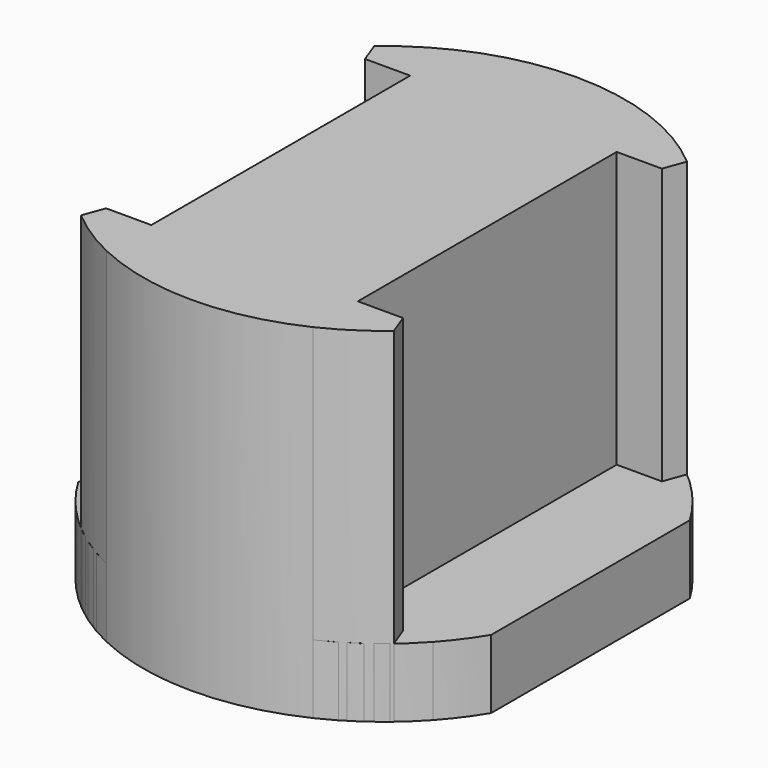
from build123d import *

# Parameters (mm, degrees)
F1_DEPTH    = 5
F0_W        = 15
F0_H        = 23.5
F2_DEPTH    = 25
F3_T1_DEPTH = 36.3750267574
F4_DEPTH    = 15


# Not quite as in the source:
# - a fillet or chamfer that OpenCascade refuses, or shapes differently, is made with other operations: its cross-section is extruded or revolved along the edge and cut away or added
# - a feature names something its author has since deleted; it is built from what else it names


with BuildPart() as f1:
    # F0 (on Top) → F1 (new body)
    with BuildSketch(Plane.XY):
        with BuildLine():
            Line((15, -9.0138781887), (15, 9.0138781887))
            ThreePointArc((15, 9.0138781887), (14.0511141288, 10.4314999755), (12.9687123493, 11.75))
            Line((12.9687123493, 11.75), (7.5, 11.75))
            Line((7.5, 11.75), (7.5, -11.75))
            Line((7.5, -11.75), (12.9687123493, -11.75))
            ThreePointArc((12.9687123493, -11.75), (14.0511141288, -10.4314999755), (15, -9.0138781887))
        make_face()
        with BuildLine():
            ThreePointArc((7.5, -15.8113883008), (10.4338758399, -14.0493499834), (12.9687123493, -11.75))
            Line((12.9687123493, -11.75), (7.5, -11.75))
            Line((7.5, -11.75), (7.5, -15.8113883008))
        make_face()
        with BuildLine():
            Line((7.5, 11.75), (12.9687123493, 11.75))
            ThreePointArc((12.9687123493, 11.75), (10.4338758399, 14.0493499834), (7.5, 15.8113883008))
            Line((7.5, 15.8113883008), (7.5, 11.75))
        make_face()
    extrude(amount=F1_DEPTH)


with BuildPart() as f1b:
    # F0 (on Top) → F1, piece 2 (new body)
    with BuildSketch(Plane.XY):
        with BuildLine():
            Line((-7.5, -11.75), (-7.5, 11.75))
            Line((-7.5, 11.75), (-12.9687123493, 11.75))
            ThreePointArc((-12.9687123493, 11.75), (-14.0511141288, 10.4314999755), (-15, 9.0138781887))
            Line((-15, 9.0138781887), (-15, -9.0138781887))
            ThreePointArc((-15, -9.0138781887), (-14.0511141288, -10.4314999755), (-12.9687123493, -11.75))
            Line((-12.9687123493, -11.75), (-7.5, -11.75))
        make_face()
        with BuildLine():
            Line((-7.5, 11.75), (-7.5, 15.8113883008))
            ThreePointArc((-7.5, 15.8113883008), (-10.4338758399, 14.0493499834), (-12.9687123493, 11.75))
            Line((-12.9687123493, 11.75), (-7.5, 11.75))
        make_face()
        with BuildLine():
            ThreePointArc((-12.9687123493, -11.75), (-10.4338758399, -14.0493499834), (-7.5, -15.8113883008))
            Line((-7.5, -15.8113883008), (-7.5, -11.75))
            Line((-7.5, -11.75), (-12.9687123493, -11.75))
        make_face()
    extrude(amount=F1_DEPTH)


with BuildPart() as f2:
    # F0 (on Top) → F2 (new body)
    with BuildSketch(Plane.XY):
        Rectangle(F0_W, F0_H)
        Polygon((-5.6291651246, 3.25), (0, 6.5), (5.6291651246, 3.25), (5.6291651246, -3.25), (0, -6.5), (-5.6291651246, -3.25), align=None, mode=Mode.SUBTRACT)
        with BuildLine():
            ThreePointArc((-12.9687123493, -11.75), (-10.4338758399, -14.0493499834), (-7.5, -15.8113883008))
            Line((-7.5, -15.8113883008), (-7.5, -11.75))
            Line((-7.5, -11.75), (-12.9687123493, -11.75))
        make_face()
        with BuildLine():
            Line((-7.5, 11.75), (-7.5, 15.8113883008))
            ThreePointArc((-7.5, 15.8113883008), (-10.4338758399, 14.0493499834), (-12.9687123493, 11.75))
            Line((-12.9687123493, 11.75), (-7.5, 11.75))
        make_face()
        with BuildLine():
            Line((7.5, 11.75), (12.9687123493, 11.75))
            ThreePointArc((12.9687123493, 11.75), (10.4338758399, 14.0493499834), (7.5, 15.8113883008))
            Line((7.5, 15.8113883008), (7.5, 11.75))
        make_face()
        with BuildLine():
            ThreePointArc((7.5, -15.8113883008), (10.4338758399, -14.0493499834), (12.9687123493, -11.75))
            Line((12.9687123493, -11.75), (7.5, -11.75))
            Line((7.5, -11.75), (7.5, -15.8113883008))
        make_face()
        with BuildLine():
            Line((7.5, 11.75), (7.5, 15.8113883008))
            ThreePointArc((7.5, 15.8113883008), (0, 17.5), (-7.5, 15.8113883008))
            Line((-7.5, 15.8113883008), (-7.5, 11.75))
            Line((-7.5, 11.75), (7.5, 11.75))
        make_face()
        with BuildLine():
            ThreePointArc((-7.5, -15.8113883008), (0, -17.5), (7.5, -15.8113883008))
            Line((7.5, -15.8113883008), (7.5, -11.75))
            Line((7.5, -11.75), (-7.5, -11.75))
            Line((-7.5, -11.75), (-7.5, -15.8113883008))
        make_face()
        Polygon((5.6291651246, 3.25), (0, 6.5), (-5.6291651246, 3.25), (-5.6291651246, -3.25), (0, -6.5), (5.6291651246, -3.25), align=None)
    extrude(amount=F2_DEPTH)

    # F3: chamfer of 2 on 4 edges, made by hand

    # F3_s2 → F3_t1 (cut)
    with BuildSketch(Plane.XY.offset(-5.6875133787)):
        with BuildLine():
            Line((-10.7571586121, -11.6749396443), (-11.3881617362, -13.3863096005))
            Line((-11.3881617362, -13.3863096005), (-11.4141285615, -13.4167353131))
            ThreePointArc((-11.4141285615, -13.4167353131), (-12.2058182488, -12.5964122224), (-12.9983551204, -11.7768571429))
            Line((-12.9983551204, -11.7768571429), (-12.9687123493, -11.71))
            ThreePointArc((-12.9687123493, -11.71), (-11.8629354807, -11.71), (-10.7571586121, -11.6349396443))
            Line((-10.7571586121, -11.6349396443), (-10.7571586121, -11.6749396443))
        make_face()
        with BuildLine():
            Line((11.3881617362, -13.3863096005), (10.7571586121, -11.6749396443))
            Line((10.7571586121, -11.6749396443), (10.7571586121, -11.6349396443))
            ThreePointArc((10.7571586121, -11.6349396443), (11.8629354807, -11.71), (12.9687123493, -11.71))
            Line((12.9687123493, -11.71), (12.9983551204, -11.7768571429))
            ThreePointArc((12.9983551204, -11.7768571429), (12.2058182488, -12.5964122224), (11.4141285615, -13.4167353131))
            Line((11.4141285615, -13.4167353131), (11.3881617362, -13.3863096005))
        make_face()
        with BuildLine():
            Line((10.7571586121, 11.6749396443), (11.3881617362, 13.3863096005))
            Line((11.3881617362, 13.3863096005), (11.4141285615, 13.4167353131))
            ThreePointArc((11.4141285615, 13.4167353131), (12.2058182488, 12.5964122224), (12.9983551204, 11.7768571429))
            Line((12.9983551204, 11.7768571429), (12.9687123493, 11.71))
            ThreePointArc((12.9687123493, 11.71), (11.8629354807, 11.71), (10.7571586121, 11.6349396443))
            Line((10.7571586121, 11.6349396443), (10.7571586121, 11.6749396443))
        make_face()
        with BuildLine():
            Line((-11.3881617362, 13.3863096005), (-10.7571586121, 11.6749396443))
            Line((-10.7571586121, 11.6749396443), (-10.7571586121, 11.6349396443))
            ThreePointArc((-10.7571586121, 11.6349396443), (-11.8629354807, 11.71), (-12.9687123493, 11.71))
            Line((-12.9687123493, 11.71), (-12.9983551204, 11.7768571429))
            ThreePointArc((-12.9983551204, 11.7768571429), (-12.2058182488, 12.5964122224), (-11.4141285615, 13.4167353131))
            Line((-11.4141285615, 13.4167353131), (-11.3881617362, 13.3863096005))
        make_face()
    extrude(amount=F3_T1_DEPTH, mode=Mode.SUBTRACT)

    # F0 (on Top) → F4 (cut)
    with BuildSketch(Plane.XY):
        Polygon((5.6291651246, 3.25), (0, 6.5), (-5.6291651246, 3.25), (-5.6291651246, -3.25), (0, -6.5), (5.6291651246, -3.25), align=None)
    extrude(amount=F4_DEPTH, mode=Mode.SUBTRACT)


solid = Compound([f1.part, f1b.part, f2.part])
